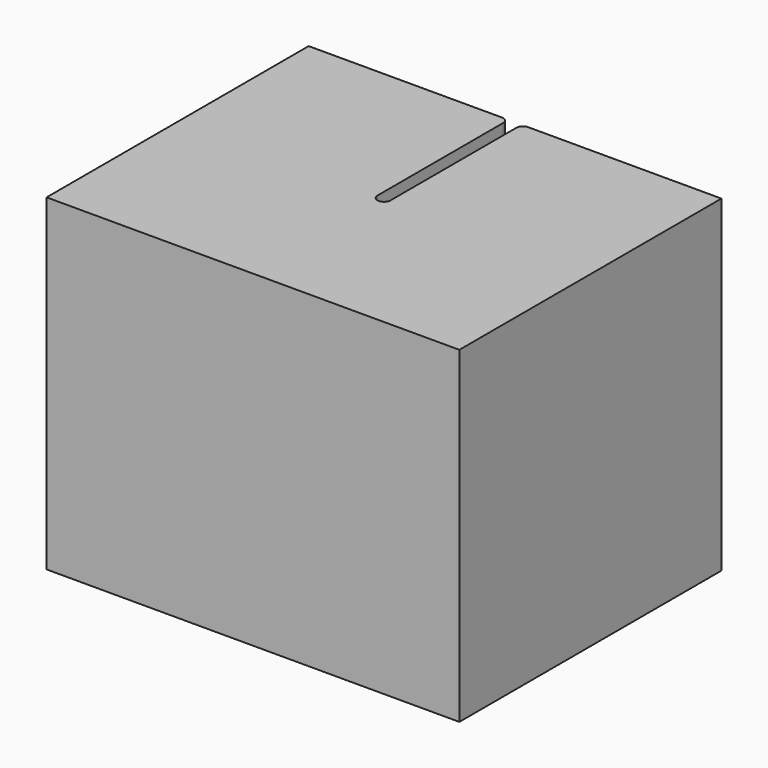
from build123d import *

# Parameters (mm, degrees)
F1_DEPTH = 10
F2_R     = 1
F3_DEPTH = 6.2


# Not quite as in the source:
# - ends of sketch curves that miss each other by under 0.0002 mm in the source are joined


with BuildPart() as f1:
    # F0 (on Top) → F1 (new body)
    with BuildSketch(Plane.XY):
        with BuildLine():
            Line((-0.3999973293, 5), (-6.2999973293, 5))
            Line((-6.2999973293, 5), (-6.2999973293, -5))
            Line((-6.2999973293, -5), (6.3, -5))
            Line((6.3, -5), (6.3, 5))
            Line((6.3, 5), (0.4, 5))
            ThreePointArc((0.4, 5), (0.2585786438, 4.9414213562), (0.2, 4.8))
            Line((0.2, 4.8), (0.2, 0))
            ThreePointArc((0.2, 0), (0.1414213562, -0.1414213562), (0, -0.2))
            ThreePointArc((0, -0.2), (-0.1414186856, -0.1414213562), (-0.1999973293, 0))
            Line((-0.1999973293, 0), (-0.1999973293, 4.8))
            ThreePointArc((-0.1999973293, 4.8), (-0.2585759731, 4.9414213562), (-0.3999973293, 5))
        make_face()
    extrude(amount=F1_DEPTH)

    # F2 (on face) → F3 (cut)
    with BuildSketch(Plane(origin=(-6.2999973293, 0, 0), x_dir=(0, -1, 0), z_dir=(-1, 0, 0))):
        with Locations((-3, 5)):
            Circle(F2_R)
    extrude(amount=-F3_DEPTH, mode=Mode.SUBTRACT)


solid = f1.part
